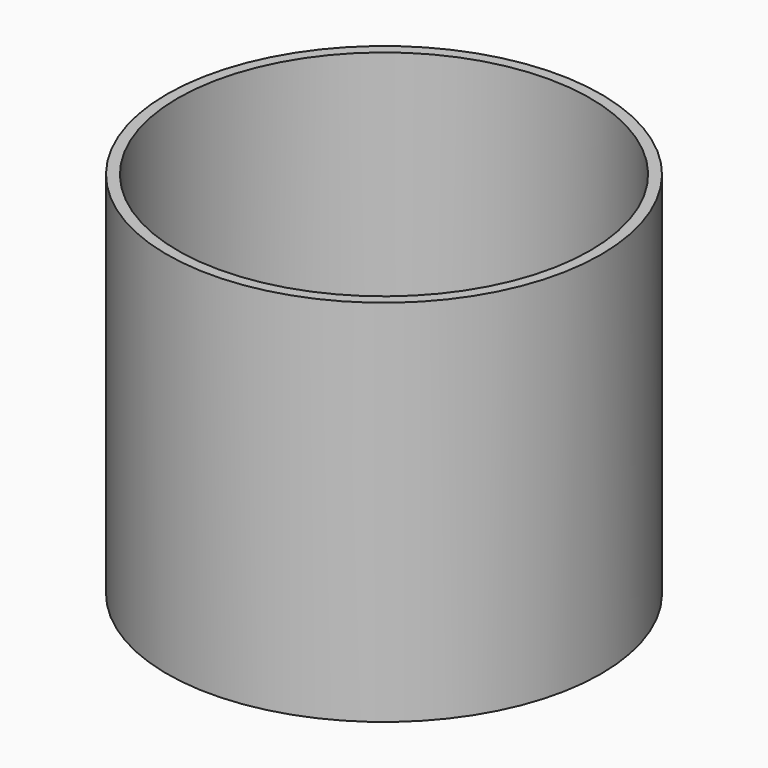
from build123d import *

# Parameters (mm, degrees)
F0_R     = 63.5
F0_R_2   = 44.45
F1_DEPTH = 6.35
F2_R     = 63.5
F2_R_2   = 60.325
F3_DEPTH = 101.6


# Not quite as in the source:
# - a length typed as a fraction of an inch, garbled in the dataset ("3 / 203.2 mm" for 3/8 in), is restored


with BuildPart() as f1:
    # F0 (on Top) → F1 (new body)
    with BuildSketch(Plane.XY):
        Circle(F0_R)
        Circle(F0_R_2, mode=Mode.SUBTRACT)
    extrude(amount=F1_DEPTH)

    # F2 (on face) → F3 (join)
    with BuildSketch(Plane.XY.offset(6.35)):
        Circle(F2_R)
        Circle(F2_R_2, mode=Mode.SUBTRACT)
    extrude(amount=F3_DEPTH)


solid = f1.part
